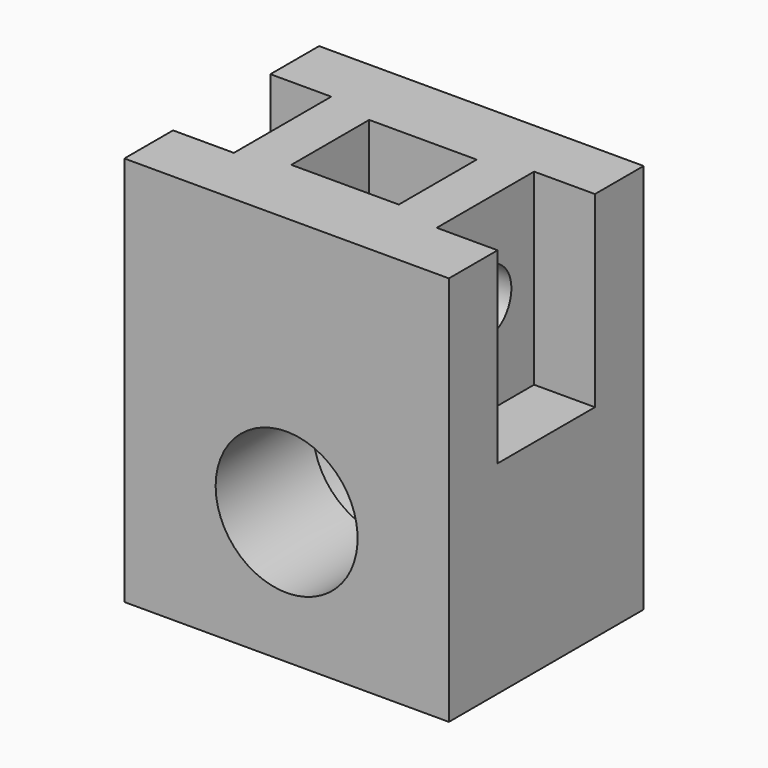
from build123d import *

# Parameters (mm, degrees)
F1_DEPTH      = 9.25
F2_R          = 1.6
F3_DEPTH      = 13.001
F4_W          = 16
F4_H          = 10
F5_DEPTH      = 6
F6_DEPTH      = 6
F7_R          = 3.5
F8_DEPTH      = 12.001
F9_R          = 5.5
F10_DEPTH     = 6
F11_W         = 5.3
F11_H         = 4.8
F12_DEPTH     = 7
F13_TEXT_SIZE = 2.9944814742
F14_DEPTH     = 1


# Not quite as in the source:
# - Text() gives the source's letters only with a copy of the font that has no kerning and outlines rounded to 1/6400 em; it was checked with that copy


with BuildPart() as f1:
    # F0 (on Top) → F1 (new body)
    with BuildSketch(Plane.XY):
        Polygon((8, 6), (-8, 6), (-8, 3), (-5, 3), (-5, -3), (-8, -3), (-8, -6), (8, -6), (8, -3), (5, -3), (5, 3), (8, 3), align=None)
    extrude(amount=F1_DEPTH)

    # F2 (on face) → F3 (cut, through all)
    with BuildSketch(Plane.YZ.offset(5)):
        with Locations((0, 4.75)):
            Circle(F2_R)
    extrude(amount=-F3_DEPTH, mode=Mode.SUBTRACT)

    # F4 (on Front) → F5 (join)
    with BuildSketch(Plane.XZ):
        with Locations((0, -5)):
            Rectangle(F4_W, F4_H)
    extrude(amount=F5_DEPTH)

    # F4 (on Front) → F6 (join)
    with BuildSketch(Plane.XZ):
        with Locations((0, -5)):
            Rectangle(F4_W, F4_H)
    extrude(amount=-F6_DEPTH)

    # F7 (on face) → F8 (cut, through all)
    with BuildSketch(Plane(origin=(0, 6, 0), x_dir=(-1, 0, 0), z_dir=(0, 1, 0))):
        with Locations((0, -3.5)):
            Circle(F7_R)
    extrude(amount=-F8_DEPTH, mode=Mode.SUBTRACT)

    # F9 (on face) → F10 (cut)
    with BuildSketch(Plane(origin=(0, 6, 0), x_dir=(-1, 0, 0), z_dir=(0, 1, 0))):
        with Locations((0, -3.5)):
            Circle(F9_R)
    extrude(amount=-F10_DEPTH, mode=Mode.SUBTRACT)

    # F11 (on face) → F12 (cut)
    with BuildSketch(Plane.XY.offset(9.25)):
        Rectangle(F11_W, F11_H)
    extrude(amount=-F12_DEPTH, mode=Mode.SUBTRACT)

    # F13 (on face) → F14 (cut)
    with BuildSketch(Plane(origin=(0, 6, 0), x_dir=(-1, 0, 0), z_dir=(0, 1, 0))):
        with Locations((-7.0197196183, 4.7044772655)):
            Text('O-339-2-B', F13_TEXT_SIZE, font='Open Sans', text_align=(TextAlign.LEFT, TextAlign.BOTTOM))
    extrude(amount=-F14_DEPTH, mode=Mode.SUBTRACT)


solid = f1.part
